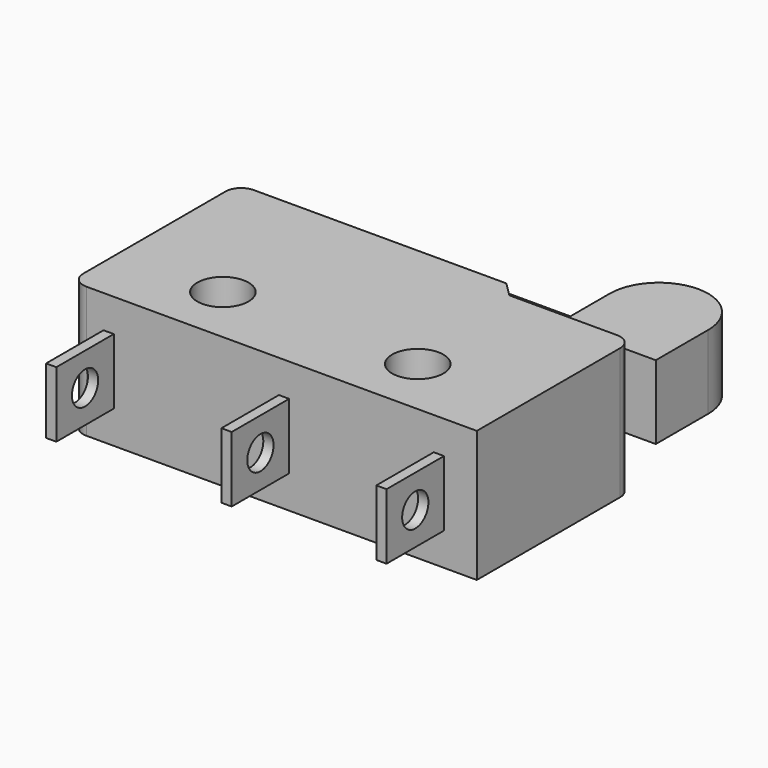
from build123d import *

# Parameters (mm, degrees)
F0_W     = 0.5
F0_H     = 3.5
F0_R     = 1.25
F1_DEPTH = 6.4
F2_W     = 25.4
F2_H     = 1.4
F2_W_2   = 3.5
F2_H_2   = 1.6
F2_R     = 0.8
F3_DEPTH = 19.8
F4_R     = 0.762


with BuildPart() as f1:
    # F0 (on Top) → F1 (new body)
    with BuildSketch(Plane.XY):
        with Locations((4.1668843009, -11.25)):
            Rectangle(F0_W, F0_H)
        with Locations((-3.3831156991, -11.25)):
            Rectangle(F0_W, F0_H)
        with Locations((-11.9331156991, -11.25)):
            Rectangle(F0_W, F0_H)
        with BuildLine():
            Line((-10.6081156991, 0.7), (-9.8143656991, 0.7))
            Line((-9.8143656991, 0.7), (-9.8143656991, 1.101979753))
            ThreePointArc((-9.8143656991, 1.101979753), (-9.7252470071, 1.317131308), (-9.5100954521, 1.40625))
            Line((-9.5100954521, 1.40625), (6.0168843009, 1.40625))
            Line((6.0168843009, 1.40625), (6.0168843009, 2.2))
            Line((6.0168843009, 2.2), (6.0168843009, 4.6))
            ThreePointArc((6.0168843009, 4.6), (3.6168843009, 7), (1.2168843009, 4.6))
            Line((1.2168843009, 4.6), (1.2168843009, 2.2))
            Line((1.2168843009, 2.2), (-9.5100954521, 2.2))
            ThreePointArc((-9.5100954521, 2.2), (-10.2865130147, 1.8783973155), (-10.6081156991, 1.101979753))
            Line((-10.6081156991, 1.101979753), (-10.6081156991, 0.7))
        make_face()
        with BuildLine():
            Line((6.0168843009, 0), (0, 0))
            Line((0, 0), (-0.7, 0.7))
            Line((-0.7, 0.7), (-5.9126656991, 0.7))
            ThreePointArc((-5.9126656991, 0.7), (-6.5935156991, 1.38085), (-7.2743656991, 0.7))
            Line((-7.2743656991, 0.7), (-9.8143656991, 0.7))
            Line((-9.8143656991, 0.7), (-10.6081156991, 0.7))
            Line((-10.6081156991, 0.7), (-13.7831156991, 0.7))
            Line((-13.7831156991, 0.7), (-13.7831156991, -9.5))
            Line((-13.7831156991, -9.5), (-12.1831156991, -9.5))
            Line((-12.1831156991, -9.5), (-11.6831156991, -9.5))
            Line((-11.6831156991, -9.5), (-3.6331156991, -9.5))
            Line((-3.6331156991, -9.5), (-3.1331156991, -9.5))
            Line((-3.1331156991, -9.5), (3.9168843009, -9.5))
            Line((3.9168843009, -9.5), (4.4168843009, -9.5))
            Line((4.4168843009, -9.5), (6.0168843009, -9.5))
            Line((6.0168843009, -9.5), (6.0168843009, 0))
        make_face()
        with Locations((-8.6831156991, -6.6)):
            Circle(F0_R, mode=Mode.SUBTRACT)
        with Locations((0.8168843009, -6.6)):
            Circle(F0_R, mode=Mode.SUBTRACT)
    extrude(amount=F1_DEPTH)

    # F2 (on face) → F3 (cut, through all)
    with BuildSketch(Plane(origin=(-13.7831156991, 0, 0), x_dir=(0, -1, 0), z_dir=(-1, 0, 0))):
        with Locations((-13.4, 0.7)):
            Rectangle(F2_W, F2_H)
        with Locations((-13.4, 5.7)):
            Rectangle(F2_W, F2_H)
        with Locations((11.25, 0.8)):
            Rectangle(F2_W_2, F2_H_2)
        with Locations((11.25, 5.6)):
            Rectangle(F2_W_2, F2_H_2)
        with Locations((11.25, 3.2)):
            Circle(F2_R)
    extrude(amount=-F3_DEPTH, mode=Mode.SUBTRACT)

    # F4
    f4_edges = [f1.edges().sort_by_distance(p)[0] for p in [
        (-13.783116, -9.5, 3.2),
        (6.016884, 0, 3.2),
        (-13.783116, 0.7, 3.2),
    ]]
    fillet(f4_edges, radius=F4_R)


solid = f1.part
